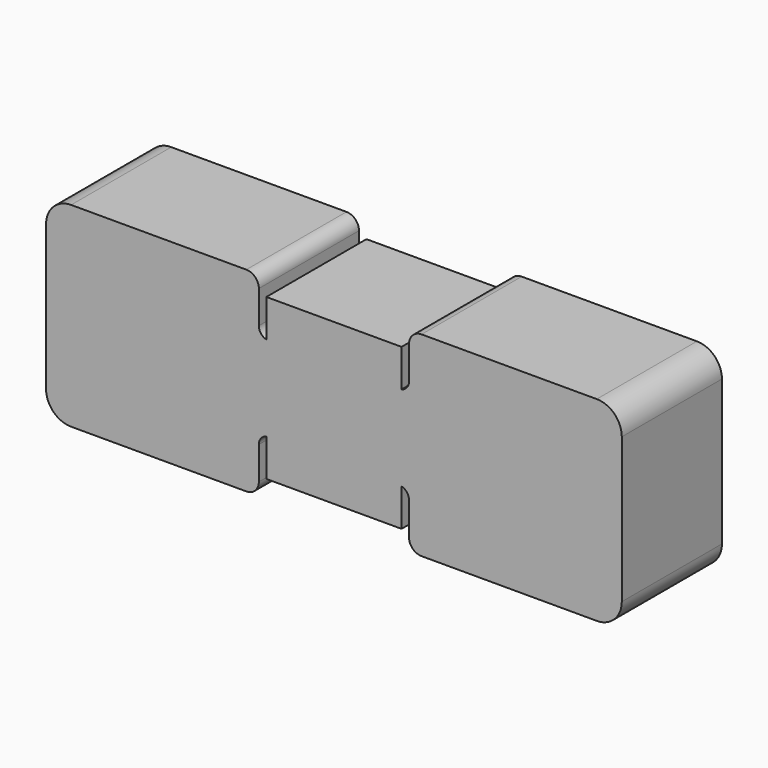
from build123d import *

# Parameters (mm, degrees)
F1_DEPTH    = 12.7
F2_R        = 2.54
F3_R        = 1.27
F4_T1_DEPTH = 12.7


# Not quite as in the source:
# - a fillet or chamfer that OpenCascade refuses, or shapes differently, is made with other operations: its cross-section is extruded or revolved along the edge and cut away or added


with BuildPart() as f1:
    # F0 (on Front) → F1 (new body)
    with BuildSketch(Plane.XZ):
        Polygon((-29.21, 0), (0, 0), (0, 8.128), (-6.858, 8.128), (-6.8540549837, 4.3214331381), (-7.62, 4.3214331381), (-7.62, 9.906), (-29.21, 9.906), align=None)
    extrude(amount=F1_DEPTH)

    # F2
    f2_edges = [f1.edges().sort_by_distance(p)[0] for p in [
        (-29.21, -6.35, 9.906),
    ]]
    fillet(f2_edges, radius=F2_R)

    # F3
    f3_edges = [f1.edges().sort_by_distance(p)[0] for p in [
        (-7.62, -6.35, 9.906),
    ]]
    fillet(f3_edges, radius=F3_R)

    # F4: fillet of radius 1.016 on 1 edges, made by hand

    # F4_s2 → F4_t1 (join)
    with BuildSketch(Plane.XZ):
        with BuildLine():
            ThreePointArc((-7.62, 5.306181078), (-7.4059700317, 4.6824022163), (-6.8540549837, 4.3214331381))
            Line((-6.8540549837, 4.3214331381), (-7.62, 4.3214331381))
            Line((-7.62, 4.3214331381), (-7.62, 5.306181078))
        make_face()
    extrude(amount=F4_T1_DEPTH)

    # F5: F1 across face


with BuildPart() as f1_1:
    add(f1.part)
    add(f1.part.mirror(Plane(origin=(-14.605, -6.35, 0), x_dir=(1, 0, 0), z_dir=(0, 0, -1))))

    # F6: F1 across face


with BuildPart() as f1_2:
    add(f1_1.part)
    add(f1_1.part.mirror(Plane(origin=(0, -6.35, 0), x_dir=(0, 1, 0), z_dir=(1, 0, 0))))


solid = f1_2.part
